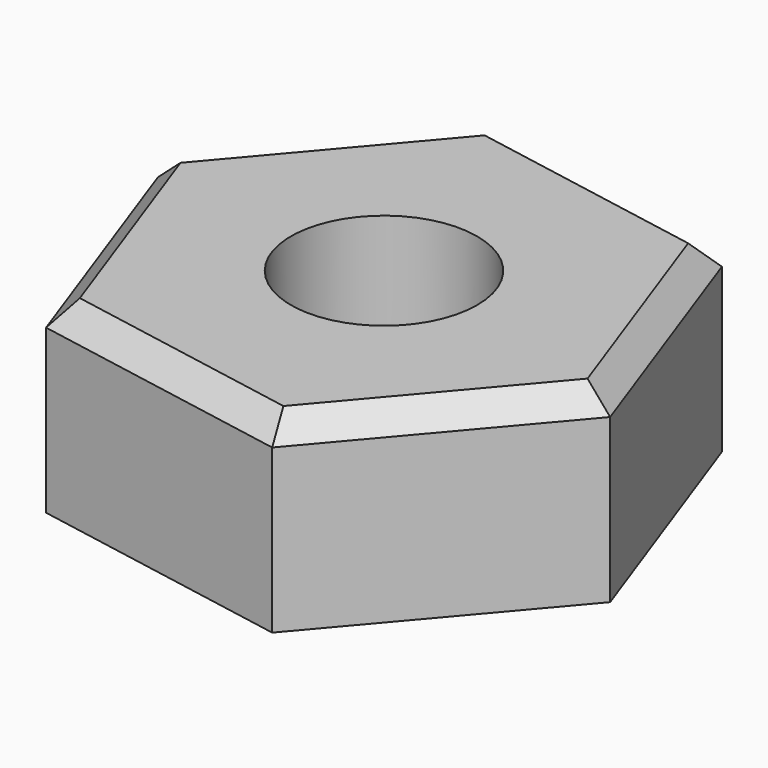
from build123d import *

# Parameters (mm, degrees)
F3_DEPTH = 4
F4_R     = 2
F5_DEPTH = 4
F6_SIZE  = 0.5


# Not quite as in the source:
# - the program builds the solid bodies; features that only make, move or delete a surface that nothing else refers to are left out


with BuildPart() as f3:
    # F2 (on Top) → F3 (new body)
    with BuildSketch(Plane.XY):
        Polygon((5.6807082187, -1.0309643387), (3.7331954171, 4.4041554595), (-1.9475128016, 5.4351197982), (-5.6807082187, 1.0309643387), (-3.7331954171, -4.4041554595), (1.9475128016, -5.4351197982), align=None)
    extrude(amount=-F3_DEPTH)

    # F4 (on face) → F5 (cut)
    with BuildSketch(Plane(origin=(0, 0, -4), x_dir=(1, 0, 0), z_dir=(0, 0, -1))):
        Circle(F4_R)
    extrude(amount=-F5_DEPTH, mode=Mode.SUBTRACT)

    # F6
    f6_edges = [f3.edges().sort_by_distance(p)[0] for p in [
        (-0.892841, -4.919638, 0),
        (3.814111, -3.233042, 0),
        (4.706952, 1.686596, 0),
        (0.892841, 4.919638, 0),
        (-3.814111, 3.233042, 0),
        (-4.706952, -1.686596, 0),
    ]]
    chamfer(f6_edges, length=F6_SIZE)


solid = f3.part
